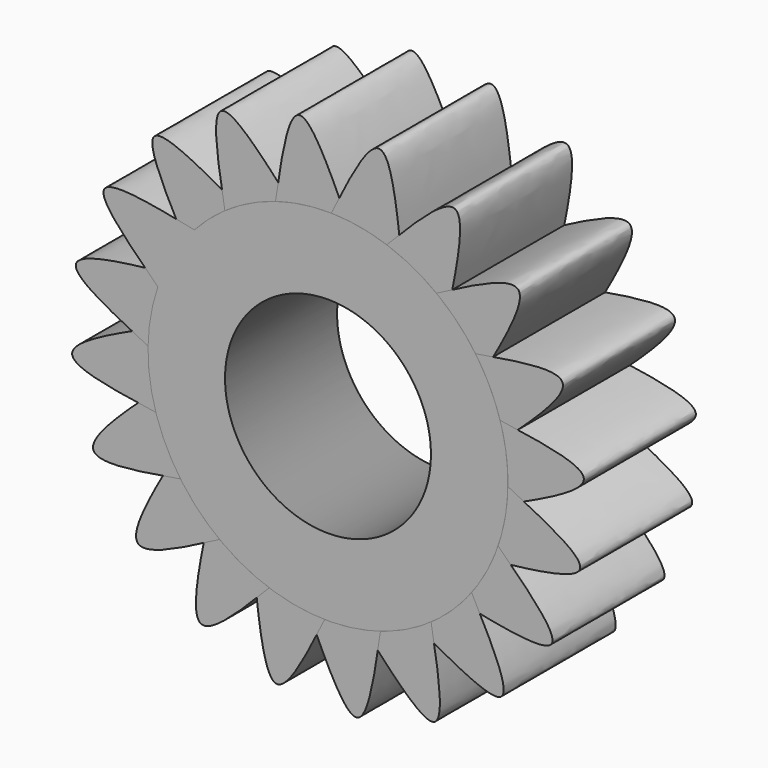
from build123d import *

# Parameters (mm, degrees)
F1_DEPTH = 50.8
F2_R     = 37.3949745599
F3_DEPTH = 131.5738484263
F4_COUNT = 20


with BuildPart() as f1:
    # F0 (on Front) → F1 (new body)
    with BuildSketch(Plane.XZ):
        with BuildLine():
            ThreePointArc((-52.1067092021, 39.3258134379), (-20.7369569457, -61.8999787), (65.2811515403, 0))
            ThreePointArc((65.2811515403, 0), (32.7004129698, 56.5005463516), (-32.5207916763, 56.6041240121))
            ThreePointArc((-32.5207916763, 56.6041240121), (-43.1866701692, 48.9544713598), (-52.1067092021, 39.3258134379))
        make_face()
        with BuildLine():
            ThreePointArc((-52.1067092021, 39.3258134379), (-43.1866701692, 48.9544713598), (-32.5207916763, 56.6041240121))
            add(Edge.make_bspline(
                [(-52.1067092021, 39.3258134379), (-59.1070799278, 52.6430142405), (-73.1757813138, 79.5063320218), (-46.1779112268, 64.2979778348), (-32.5207916763, 56.6041240121)],
                knots=[0, 0, 0, 0, 0.4948788084, 1, 1, 1, 1], degree=3))
        make_face()
    extrude(amount=F1_DEPTH)

    # F2 (on face) → F3 (cut)
    with BuildSketch(Plane.XZ.offset(50.8)):
        Circle(F2_R)
    extrude(amount=-F3_DEPTH, mode=Mode.SUBTRACT)


with BuildPart() as f4_1:
    # F4: instance of F1
    add(f1.part.rotate(Axis((0, 0, 0), (0, 1, 0)), 1 * 360 / F4_COUNT))


with BuildPart() as f4_2:
    # F4: instance of F1
    add(f1.part.rotate(Axis((0, 0, 0), (0, 1, 0)), 2 * 360 / F4_COUNT))


with BuildPart() as f4_3:
    # F4: instance of F1
    add(f1.part.rotate(Axis((0, 0, 0), (0, 1, 0)), 3 * 360 / F4_COUNT))


with BuildPart() as f4_4:
    # F4: instance of F1
    add(f1.part.rotate(Axis((0, 0, 0), (0, 1, 0)), 4 * 360 / F4_COUNT))


with BuildPart() as f4_5:
    # F4: instance of F1
    add(f1.part.rotate(Axis((0, 0, 0), (0, 1, 0)), 5 * 360 / F4_COUNT))


with BuildPart() as f4_6:
    # F4: instance of F1
    add(f1.part.rotate(Axis((0, 0, 0), (0, 1, 0)), 6 * 360 / F4_COUNT))


with BuildPart() as f4_7:
    # F4: instance of F1
    add(f1.part.rotate(Axis((0, 0, 0), (0, 1, 0)), 7 * 360 / F4_COUNT))


with BuildPart() as f4_8:
    # F4: instance of F1
    add(f1.part.rotate(Axis((0, 0, 0), (0, 1, 0)), 8 * 360 / F4_COUNT))


with BuildPart() as f4_9:
    # F4: instance of F1
    add(f1.part.rotate(Axis((0, 0, 0), (0, 1, 0)), 9 * 360 / F4_COUNT))


with BuildPart() as f4_10:
    # F4: instance of F1
    add(f1.part.rotate(Axis((0, 0, 0), (0, 1, 0)), 10 * 360 / F4_COUNT))


with BuildPart() as f4_11:
    # F4: instance of F1
    add(f1.part.rotate(Axis((0, 0, 0), (0, 1, 0)), 11 * 360 / F4_COUNT))


with BuildPart() as f4_12:
    # F4: instance of F1
    add(f1.part.rotate(Axis((0, 0, 0), (0, 1, 0)), 12 * 360 / F4_COUNT))


with BuildPart() as f4_13:
    # F4: instance of F1
    add(f1.part.rotate(Axis((0, 0, 0), (0, 1, 0)), 13 * 360 / F4_COUNT))


with BuildPart() as f4_14:
    # F4: instance of F1
    add(f1.part.rotate(Axis((0, 0, 0), (0, 1, 0)), 14 * 360 / F4_COUNT))


with BuildPart() as f4_15:
    # F4: instance of F1
    add(f1.part.rotate(Axis((0, 0, 0), (0, 1, 0)), 15 * 360 / F4_COUNT))


with BuildPart() as f4_16:
    # F4: instance of F1
    add(f1.part.rotate(Axis((0, 0, 0), (0, 1, 0)), 16 * 360 / F4_COUNT))


with BuildPart() as f4_17:
    # F4: instance of F1
    add(f1.part.rotate(Axis((0, 0, 0), (0, 1, 0)), 17 * 360 / F4_COUNT))


with BuildPart() as f4_18:
    # F4: instance of F1
    add(f1.part.rotate(Axis((0, 0, 0), (0, 1, 0)), 18 * 360 / F4_COUNT))


with BuildPart() as f4_19:
    # F4: instance of F1
    add(f1.part.rotate(Axis((0, 0, 0), (0, 1, 0)), 19 * 360 / F4_COUNT))


solid = Compound([f1.part, f4_1.part, f4_2.part, f4_3.part, f4_4.part, f4_5.part, f4_6.part, f4_7.part, f4_8.part, f4_9.part, f4_10.part, f4_11.part, f4_12.part, f4_13.part, f4_14.part, f4_15.part, f4_16.part, f4_17.part, f4_18.part, f4_19.part])
